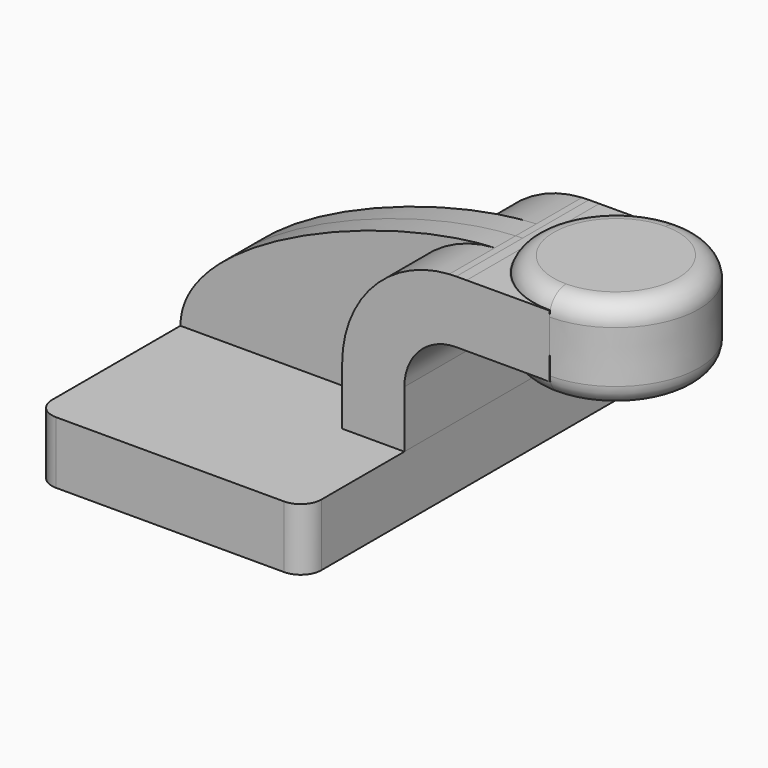
from build123d import *

# Parameters (mm, degrees)
F1_DEPTH = 63.5
F2_DEPTH = 25.4
F3_DEPTH = 7.9375
F5_F1_R  = 6.35
F5_F2_R  = 6.35
F5_F3_R  = 6.35
F5_F4_R  = 6.35


# Not quite as in the source:
# - a fillet or chamfer that OpenCascade refuses, or shapes differently, is made with other operations: its cross-section is extruded or revolved along the edge and cut away or added
# - a feature names something its author has since deleted; it is built from what else it names


with BuildPart() as f1:
    # F0 (on Front) → F1 (new body, symmetric)
    with BuildSketch(Plane.XZ):
        Polygon((-41.275, -9.525), (41.275, -9.525), (41.275, 9.525), (22.225, 9.525), (-41.275, 9.525), align=None)
    extrude(amount=F1_DEPTH, both=True)

    # F5: fillet of radius 6.35 on 4 edges, made by hand

    # F5_f1
    f5_f1_edges = [f1.edges().sort_by_distance(p)[0] for p in [
        (-41.275, 63.5, 0),
    ]]
    fillet(f5_f1_edges, radius=F5_F1_R)

    # F5_f2
    f5_f2_edges = [f1.edges().sort_by_distance(p)[0] for p in [
        (-41.275, -63.5, 0),
    ]]
    fillet(f5_f2_edges, radius=F5_F2_R)

    # F5_f3
    f5_f3_edges = [f1.edges().sort_by_distance(p)[0] for p in [
        (41.275, -63.5, 0),
    ]]
    fillet(f5_f3_edges, radius=F5_F3_R)

    # F5_f4
    f5_f4_edges = [f1.edges().sort_by_distance(p)[0] for p in [
        (41.275, 63.5, 0),
    ]]
    fillet(f5_f4_edges, radius=F5_F4_R)


with BuildPart() as f2:
    # F0 (on Front) → F2 (new body, symmetric)
    with BuildSketch(Plane.XZ):
        with BuildLine():
            Line((22.225, 9.525), (41.275, 9.525))
            Line((41.275, 9.525), (41.275, 27.0002))
            ThreePointArc((41.275, 27.0002), (45.9246798487, 38.2255201513), (57.15, 42.8752))
            Line((57.15, 42.8752), (60.325, 42.8752))
            Line((60.325, 42.8752), (60.325, 61.9331814487))
            Line((60.325, 61.9331814487), (57.15, 61.9252))
            add(Edge.make_bspline(
                [(55.0350912904, 61.8611062726), (55.7525569536, 61.8926833879), (56.457802247, 61.9141139323), (57.15, 61.9252)],
                knots=[109.2159777355, 109.2159777355, 109.2159777355, 109.2159777355, 111.5045361635, 111.5045361635, 111.5045361635, 111.5045361635], degree=3))
            ThreePointArc((55.0350912904, 61.8611062726), (31.7175521068, 50.9364950174), (22.225, 27.0002))
            Line((22.225, 27.0002), (22.225, 9.525))
        make_face()
        Polygon((60.325, 61.9331814487), (60.325, 42.8752), (85.7848289395, 42.8752), (85.736759596, 61.9970626002), align=None)
    extrude(amount=F2_DEPTH, both=True)

    # F0 (on Front) → F4 (revolve)
    with BuildSketch(Plane.XZ):
        Polygon((85.736759596, 61.9970626002), (85.7848289395, 42.8752), (85.7968330384, 38.1), (111.125, 38.1), (111.125, 66.675), (85.725, 66.675), align=None)
    revolve(axis=Axis((85.7609165192, 0, 52.3875), (0.0025138342, 0, -0.9999968403)))

    # F5#2: fillet of radius 6.35 on 2 edges, made by hand


with BuildPart() as f3:
    # F0 (on Front) → F3 (new body, symmetric)
    with BuildSketch(Plane.XZ):
        with BuildLine():
            add(Edge.make_bspline(
                [(-41.275, 9.525), (-41.2748232273, 35.7389409039), (20.7957583833, 60.354163967), (55.0350912904, 61.8611062726)],
                knots=[0, 0, 0, 0, 109.2159777355, 109.2159777355, 109.2159777355, 109.2159777355], degree=3))
            Line((-41.275, 9.525), (22.225, 9.525))
            Line((22.225, 9.525), (22.225, 27.0002))
            ThreePointArc((22.225, 27.0002), (31.7175521068, 50.9364950174), (55.0350912904, 61.8611062726))
        make_face()
    extrude(amount=F3_DEPTH, both=True)


with BuildPart() as f5_2_tool2:
    # F5_2_s3 → F5_2_t4 (revolve)
    with BuildSketch(Plane.XZ):
        with BuildLine():
            ThreePointArc((111.125, 60.325), (109.2651280605, 64.8151280605), (104.775, 66.675))
            Line((104.775, 66.675), (111.125, 66.675))
            Line((111.125, 66.675), (111.125, 60.325))
        make_face()
    revolve(axis=Axis((85.7251605118, 0, 66.6111488138), (0.0025138342, 0, -0.9999968403)))

    split(bisect_by=Plane(origin=(85.8920676364, 0, 0.2159190969), x_dir=(0, 1, 0), z_dir=(0.9999968403, 0, 0.0025138342)), keep=Keep.TOP)

    split(bisect_by=Plane(origin=(-0.1553080404, 0, 61.7811435033), x_dir=(0, 1, 0), z_dir=(0.0025138342, 0, -0.9999968403)), keep=Keep.TOP)


with BuildPart() as f2_1:
    add(f2.part)

    # F5_2_t1: cut F5_2_tool2
    add(f5_2_tool2.part, mode=Mode.SUBTRACT)


with BuildPart() as f5_2_tool8:
    # F5_2_s9 → F5_2_t10 (revolve)
    with BuildSketch(Plane.XZ):
        with BuildLine():
            ThreePointArc((111.125, 60.325), (109.2651280605, 64.8151280605), (104.775, 66.675))
            Line((104.775, 66.675), (111.125, 66.675))
            Line((111.125, 66.675), (111.125, 60.325))
        make_face()
    revolve(axis=Axis((85.7251605118, 0, 66.6111488138), (0.0025138342, 0, -0.9999968403)))

    split(bisect_by=Plane(origin=(85.8920676364, 0, 0.2159190969), x_dir=(0, 1, 0), z_dir=(0.9999968403, 0, 0.0025138342)), keep=Keep.TOP)

    split(bisect_by=Plane(origin=(-0.1553080404, 0, 61.7811435033), x_dir=(0, 1, 0), z_dir=(-0.0025138342, 0, 0.9999968403)), keep=Keep.TOP)


with BuildPart() as f2_2:
    add(f2_1.part)

    # F5_2_t7: cut F5_2_tool8
    add(f5_2_tool8.part, mode=Mode.SUBTRACT)


with BuildPart() as f5_2_tool14:
    # F5_2_s15 → F5_2_t16 (revolve)
    with BuildSketch(Plane.XZ):
        with BuildLine():
            ThreePointArc((111.125, 60.325), (109.2651280605, 64.8151280605), (104.775, 66.675))
            Line((104.775, 66.675), (111.125, 66.675))
            Line((111.125, 66.675), (111.125, 60.325))
        make_face()
    revolve(axis=Axis((85.7251605118, 0, 66.6111488138), (0.0025138342, 0, -0.9999968403)))

    split(bisect_by=Plane(origin=(85.8920676364, 0, 0.2159190969), x_dir=(0, 1, 0), z_dir=(-0.9999968403, 0, -0.0025138342)), keep=Keep.TOP)

    split(bisect_by=Plane(origin=(-0.1553080404, 0, 61.7811435033), x_dir=(0, 1, 0), z_dir=(-0.0025138342, 0, 0.9999968403)), keep=Keep.TOP)


with BuildPart() as f2_3:
    add(f2_2.part)

    # F5_2_t13: cut F5_2_tool14
    add(f5_2_tool14.part, mode=Mode.SUBTRACT)


with BuildPart() as f5_2_tool20:
    # F5_2_s21 → F5_2_t22 (revolve)
    with BuildSketch(Plane.XZ):
        with BuildLine():
            ThreePointArc((111.125, 44.45), (109.2651280605, 39.9598719395), (104.775, 38.1))
            Line((104.775, 38.1), (111.125, 38.1))
            Line((111.125, 38.1), (111.125, 44.45))
        make_face()
    revolve(axis=Axis((85.7969930963, 0, 38.0363293896), (0.0025138342, 0, -0.9999968403)))

    split(bisect_by=Plane.XY.offset(42.8752), keep=Keep.TOP)

    split(bisect_by=Plane(origin=(85.8920676364, 0, 0.2159190969), x_dir=(0, 1, 0), z_dir=(0.9999968403, 0, 0.0025138342)), keep=Keep.TOP)


with BuildPart() as f2_4:
    add(f2_3.part)

    # F5_2_t19: cut F5_2_tool20
    add(f5_2_tool20.part, mode=Mode.SUBTRACT)


with BuildPart() as f5_2_tool26:
    # F5_2_s27 → F5_2_t28 (revolve)
    with BuildSketch(Plane.XZ):
        with BuildLine():
            ThreePointArc((111.125, 44.45), (109.2651280605, 39.9598719395), (104.775, 38.1))
            Line((104.775, 38.1), (111.125, 38.1))
            Line((111.125, 38.1), (111.125, 44.45))
        make_face()
    revolve(axis=Axis((85.7969930963, 0, 38.0363293896), (0.0025138342, 0, -0.9999968403)))

    split(bisect_by=Plane.XY.offset(42.8752), keep=Keep.BOTTOM)

    split(bisect_by=Plane(origin=(85.8920676364, 0, 0.2159190969), x_dir=(0, 1, 0), z_dir=(0.9999968403, 0, 0.0025138342)), keep=Keep.TOP)


with BuildPart() as f2_5:
    add(f2_4.part)

    # F5_2_t25: cut F5_2_tool26
    add(f5_2_tool26.part, mode=Mode.SUBTRACT)


with BuildPart() as f5_2_tool32:
    # F5_2_s33 → F5_2_t34 (revolve)
    with BuildSketch(Plane.XZ):
        with BuildLine():
            ThreePointArc((111.125, 44.45), (109.2651280605, 39.9598719395), (104.775, 38.1))
            Line((104.775, 38.1), (111.125, 38.1))
            Line((111.125, 38.1), (111.125, 44.45))
        make_face()
    revolve(axis=Axis((85.7969930963, 0, 38.0363293896), (0.0025138342, 0, -0.9999968403)))

    split(bisect_by=Plane.XY.offset(42.8752), keep=Keep.BOTTOM)

    split(bisect_by=Plane(origin=(85.8920676364, 0, 0.2159190969), x_dir=(0, 1, 0), z_dir=(-0.9999968403, 0, -0.0025138342)), keep=Keep.TOP)


with BuildPart() as f2_6:
    add(f2_5.part)

    # F5_2_t31: cut F5_2_tool32
    add(f5_2_tool32.part, mode=Mode.SUBTRACT)


solid = Compound([f1.part, f3.part, f2_6.part])
